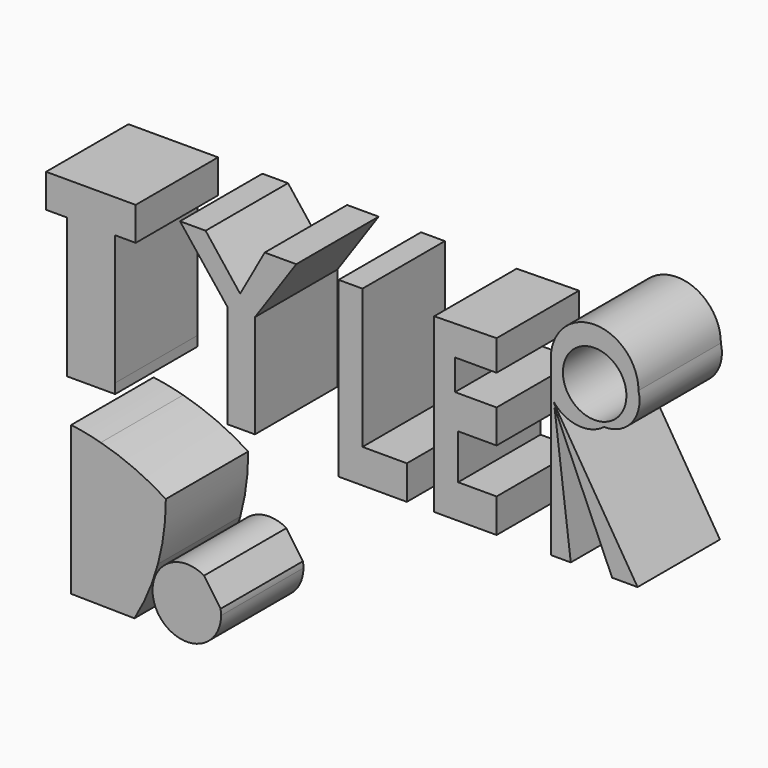
from build123d import *

# Parameters (mm, degrees)
F1_DEPTH = 25.4
F0_R     = 7.8346511006
F2_DEPTH = 25.4


# Not quite as in the source:
# - a feature names something its author has since deleted; it is built from what else it names


with BuildPart() as f1:
    # F0 (on Front) → F1 (new body)
    with BuildSketch(Plane.XZ):
        Polygon((-81.5548015942, -5.9490810307), (-81.5939936003, 26.1106837792), (-76.4789922628, 26.1106837792), (-76.4890760183, 34.3593768775), (-98.5859185457, 34.3593768775), (-98.5859185457, 26.1034145951), (-93.4866443276, 26.1034145951), (-93.4866443276, -8.3773750812), (-85.1137137568, -8.3773750812), (-81.5518330847, -8.3773750812), align=None)
    extrude(amount=F1_DEPTH)


with BuildPart() as f1b:
    # F0 (on Front) → F1, piece 2 (new body)
    with BuildSketch(Plane.XZ):
        Polygon((-53.8510866463, 19.5539519191), (-53.8510866463, -5.915214152), (-47.0775440335, -5.9069337194), (-47.0775440335, 19.5539519191), (-36.8871465325, 34.3593768775), (-44.6654930711, 34.3593768775), (-50.7271438837, 23.4395619482), (-59.2428706586, 34.3593768775), (-65.5611678958, 34.3593768775), align=None)
    extrude(amount=F1_DEPTH)


with BuildPart() as f1c:
    # F0 (on Front) → F1, piece 3 (new body)
    with BuildSketch(Plane.XZ):
        Polygon((-26.4410860837, 34.3593768775), (-26.4410860837, -5.8817063295), (-9.6088461578, -5.8611294708), (-9.6088461578, 0), (-20.5608587712, 0), (-20.5608587712, 34.3593768775), align=None)
        Polygon((-9.6088461578, -5.8611294708), (-26.4410860837, -5.8817063295), (-26.4410860837, -8.3773750812), (-9.6088461578, -8.3773750812), align=None)
    extrude(amount=F1_DEPTH)


with BuildPart() as f1d:
    # F0 (on Front) → F1, piece 4 (new body)
    with BuildSketch(Plane.XZ):
        Polygon((-2.8605444822, 34.1275193292), (-2.8605444822, -5.8528798943), (-2.8605444822, -8.3773750812), (12.5163393095, -8.3773750812), (12.5163393095, 0), (3.0234002043, 0), (3.0234002043, 11.0600087792), (12.5163393095, 11.0600087792), (12.5163393095, 19.3200614303), (2.2653094493, 19.3200614303), (2.2653094493, 26.8484186381), (12.5163393095, 26.8484186381), (12.5163393095, 34.3593768775), align=None)
    extrude(amount=F1_DEPTH)


with BuildPart() as f1e:
    # F0 (on Front) → F1, piece 5 (new body)
    with BuildSketch(Plane.XZ):
        Polygon((25.887073949, -5.817736878), (25.887073949, -8.3773750812), (30.8153238147, -8.3773750812), (26.804734222, 24.0303265492), (25.887073949, 26.1232946068), align=None)
        Polygon((41.013866663, -8.3773750812), (47.2822114825, -8.3773750812), (26.7099292009, 24.7964016527), (26.804734222, 24.0303265492), align=None)
        with BuildLine():
            Line((25.887073949, 31.4455106854), (25.887073949, 26.1232946068))
            ThreePointArc((25.887073949, 26.1232946068), (26.2634233094, 25.5641583421), (26.6804434798, 25.0346619955))
            Line((26.6804434798, 25.0346619955), (25.887073949, 31.4455106854))
        make_face()
        with BuildLine():
            Line((25.887073949, 31.4455106854), (26.6804434798, 25.0346619955))
            ThreePointArc((26.6804434798, 25.0346619955), (32.5853799721, 21.9064737064), (39.0235707164, 23.6963164061))
            ThreePointArc((39.0235707164, 23.6963164061), (45.8972704971, 26.9351735913), (47.5156493485, 34.3593768775))
            ThreePointArc((47.5156493485, 34.3593768775), (36.7013616487, 45.1736645773), (25.887073949, 34.3593768775))
            Line((25.887073949, 34.3593768775), (25.887073949, 31.4455106854))
        make_face()
        with Locations((36.7013616487, 32.2891227819)):
            Circle(F0_R, mode=Mode.SUBTRACT)
        with BuildLine():
            Line((25.887073949, 26.1232946068), (26.7099292009, 24.7964016527))
            Line((26.7099292009, 24.7964016527), (26.6804434798, 25.0346619955))
            ThreePointArc((26.6804434798, 25.0346619955), (26.2634233094, 25.5641583421), (25.887073949, 26.1232946068))
        make_face()
        Polygon((26.804734222, 24.0303265492), (26.7099292009, 24.7964016527), (25.887073949, 26.1232946068), align=None)
    extrude(amount=F1_DEPTH)


with BuildPart() as f1f:
    # F0 (on Front) → F1, piece 6 (new body)
    with BuildSketch(Plane.XZ):
        with BuildLine():
            ThreePointArc((-69.052644074, -27.0859580487), (-76.8098655757, -22.9616357633), (-85.0994422189, -20.0517493705))
            ThreePointArc((-85.0994422189, -20.0517493705), (-88.7208301281, -19.2034415659), (-92.3890024424, -18.5881461948))
            Line((-92.3890024424, -18.5881461948), (-92.3890024424, -55.2658587694))
            Line((-92.3890024424, -55.2658587694), (-76.7976269126, -55.5061623454))
            ThreePointArc((-76.7976269126, -55.5061623454), (-73.4330277562, -48.8605222286), (-70.9939883224, -41.8223302246))
            ThreePointArc((-70.9939883224, -41.8223302246), (-69.5249399969, -34.5197993576), (-69.052644074, -27.0859580487))
        make_face()
    extrude(amount=F1_DEPTH)


with BuildPart() as f1g:
    # F0 (on Front) → F1, piece 7 (new body)
    with BuildSketch(Plane.XZ):
        with BuildLine():
            Line((-70.9939883224, -44.3777080037), (-69.6910760743, -41.8223302246))
            ThreePointArc((-69.6910760743, -41.8223302246), (-71.4103560372, -44.1206987553), (-72.2607105289, -46.8621069212))
            Line((-72.2607105289, -46.8621069212), (-70.9939883224, -44.3777080037))
        make_face()
    extrude(amount=F1_DEPTH)

    # F0 (on Front) → F2 (join)
    with BuildSketch(Plane.XZ):
        with BuildLine():
            Line((-55.5599836481, -46.5320129656), (-59.6358900865, -40.6576858918))
            ThreePointArc((-59.6358900865, -40.6576858918), (-64.8572673415, -39.5669335136), (-69.6910760743, -41.8223302246))
            Line((-69.6910760743, -41.8223302246), (-70.9939883224, -44.3777080037))
            Line((-70.9939883224, -44.3777080037), (-72.2607105289, -46.8621069212))
            ThreePointArc((-72.2607105289, -46.8621069212), (-70.4274922661, -53.3003248587), (-64.4852485065, -56.3827068131))
            ThreePointArc((-64.4852485065, -56.3827068131), (-58.1287611445, -54.1385093801), (-55.4388398996, -47.9574352503))
            ThreePointArc((-55.4388398996, -47.9574352503), (-55.4691803286, -47.2421547987), (-55.5599836481, -46.5320129656))
        make_face()
    extrude(amount=F2_DEPTH)


solid = Compound([f1.part, f1b.part, f1c.part, f1d.part, f1e.part, f1f.part, f1g.part])
